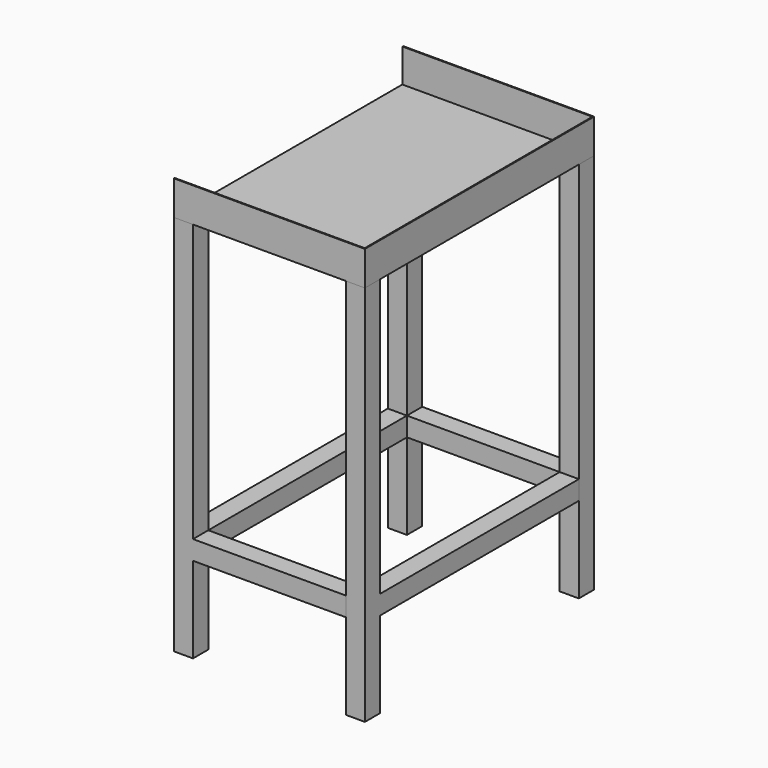
from build123d import *

# Parameters (mm, degrees)
F0_W      = 40
F0_H      = 40
F1_DEPTH  = 800
F2_W      = 400
F2_H      = 600
F3_DEPTH  = 2
F5_DEPTH  = 70
F6_W      = 40
F6_H      = 40
F7_DEPTH  = 520
F8_W      = 40
F8_H      = 40
F9_DEPTH  = 320
F10_W     = 40
F10_H     = 40
F11_DEPTH = 520
F12_W     = 40
F12_H     = 40
F13_DEPTH = 320


with BuildPart() as f1:
    # F0 (on Top) → F1 (new body)
    with BuildSketch(Plane.XY):
        with Locations((-180, 280)):
            Rectangle(F0_W, F0_H)
    extrude(amount=F1_DEPTH)

    # F2 (on face) → F3 (join)
    with BuildSketch(Plane.XY.offset(800)):
        Rectangle(F2_W, F2_H)
    extrude(amount=F3_DEPTH)

    # F4 (on face) → F5 (join)
    with BuildSketch(Plane.XY.offset(802)):
        Polygon((200, 300), (-200, 300), (-200, 298), (198, 298), (198, -298), (-200, -298), (-200, -300), (200, -300), align=None)
    extrude(amount=F5_DEPTH)

    # F6 (on face) → F7 (join, through all)
    with BuildSketch(Plane.XZ.offset(-260)):
        with Locations((-180, 200)):
            Rectangle(F6_W, F6_H)
    extrude(amount=F7_DEPTH)


with BuildPart() as f1b:
    # F0 (on Top) → F1, piece 2 (new body)
    with BuildSketch(Plane.XY):
        with Locations((-180, -280)):
            Rectangle(F0_W, F0_H)
    extrude(amount=F1_DEPTH)

    # F8 (on face) → F9 (join, through all)
    with BuildSketch(Plane.YZ.offset(-160)):
        with Locations((-280, 200)):
            Rectangle(F8_W, F8_H)
    extrude(amount=F9_DEPTH)


with BuildPart() as f1c:
    # F0 (on Top) → F1, piece 3 (new body)
    with BuildSketch(Plane.XY):
        with Locations((180, 280)):
            Rectangle(F0_W, F0_H)
    extrude(amount=F1_DEPTH)

    # F12 (on face) → F13 (join, through all)
    with BuildSketch(Plane(origin=(160, 0, 0), x_dir=(0, -1, 0), z_dir=(-1, 0, 0))):
        with Locations((-280, 200)):
            Rectangle(F12_W, F12_H)
    extrude(amount=F13_DEPTH)


with BuildPart() as f1d:
    # F0 (on Top) → F1, piece 4 (new body)
    with BuildSketch(Plane.XY):
        with Locations((180, -280)):
            Rectangle(F0_W, F0_H)
    extrude(amount=F1_DEPTH)

    # F10 (on face) → F11 (join, through all)
    with BuildSketch(Plane(origin=(0, -260, 0), x_dir=(-1, 0, 0), z_dir=(0, 1, 0))):
        with Locations((-180, 200)):
            Rectangle(F10_W, F10_H)
    extrude(amount=F11_DEPTH)


solid = Compound([f1.part, f1b.part, f1c.part, f1d.part])
